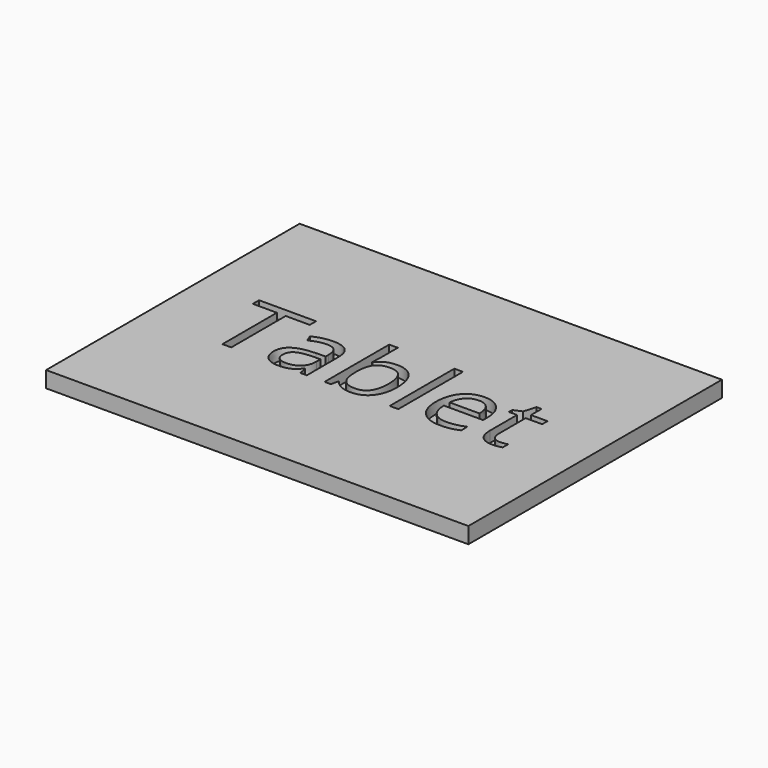
from build123d import *

# Parameters (mm, degrees)
F0_W         = 246.38
F0_H         = 184.912
F1_DEPTH     = 9.398
F2_TEXT_SIZE = 62.0273948811
F3_DEPTH     = 6.35


# Not quite as in the source:
# - Text() gives the source's letters only with a copy of the font that has no kerning and outlines rounded to 1/6400 em; it was checked with that copy


with BuildPart() as f1:
    # F0 (on Top) → F1 (new body)
    with BuildSketch(Plane.XY):
        with Locations((123.19, 92.456)):
            Rectangle(F0_W, F0_H)
    extrude(amount=F1_DEPTH)

    # F2 (on face) → F3 (cut)
    with BuildSketch(Plane.XY.offset(9.398)):
        with Locations((32.2229486946, 70.1261378428)):
            Text('Tablet', F2_TEXT_SIZE, font='Open Sans', text_align=(TextAlign.LEFT, TextAlign.BOTTOM))
    extrude(amount=-F3_DEPTH, mode=Mode.SUBTRACT)


solid = f1.part
